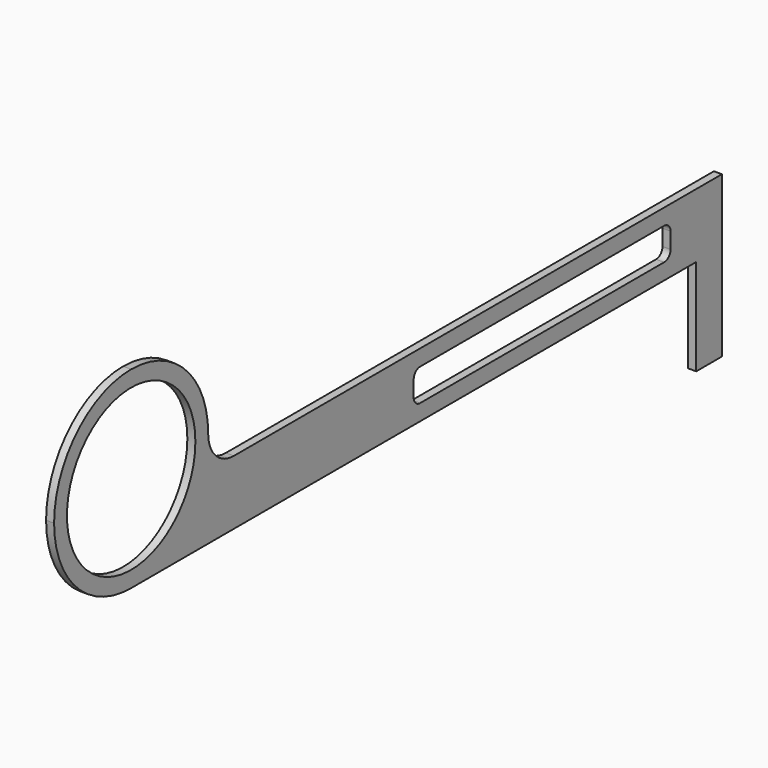
from build123d import *

# Parameters (mm, degrees)
F1_DEPTH = 1.5875
F2_R     = 19.04999
F3_R     = 6.35
F4_R     = 15.875
F5_DEPTH = 25.4
F6_W     = 63.5
F6_H     = 6.35
F7_DEPTH = 25.4
F8_R     = 1.5875


# Not quite as in the source:
# - a fillet or chamfer is up to 0.001 mm smaller than in the source, because OpenCascade refuses the exact size


with BuildPart() as f1:
    # F0 (on Right) → F1 (new body)
    with BuildSketch(Plane.YZ):
        Polygon((-63.1363113923, 43.5325428513), (-101.2363113923, 43.5325428513), (-101.2363113923, 5.4325428513), (57.5136886077, 5.4325428513), (57.5136886077, -13.6174602094), (63.8636886077, -13.6174602094), (63.8636886077, 18.1325428513), (-63.1363113923, 18.1325428513), align=None)
    extrude(amount=F1_DEPTH)

    # F2 (radius 19.05 in the source; OpenCascade refuses exactly that, so slightly less here)
    f2_edges = [f1.edges().sort_by_distance(p)[0] for p in [
        (0.79375, -63.136311, 43.532543),
        (0.79375, -101.236311, 43.532543),
        (0.79375, -101.236311, 5.432543),
    ]]
    fillet(f2_edges, radius=F2_R)

    # F3
    f3_edges = [f1.edges().sort_by_distance(p)[0] for p in [
        (0.79375, -63.136311, 18.132543),
    ]]
    fillet(f3_edges, radius=F3_R)

    # F4 (on face) → F5 (cut)
    with BuildSketch(Plane.YZ.offset(1.5875)):
        with Locations((-82.1863113923, 24.4825428513)):
            Circle(F4_R)
    extrude(amount=-F5_DEPTH, mode=Mode.SUBTRACT)

    # F6 (on face) → F7 (cut)
    with BuildSketch(Plane.YZ.offset(1.5875)):
        with Locations((19.4136886077, 11.7825428513)):
            Rectangle(F6_W, F6_H)
    extrude(amount=-F7_DEPTH, mode=Mode.SUBTRACT)

    # F8
    f8_edges = [f1.edges().sort_by_distance(p)[0] for p in [
        (0.79375, -12.336311, 14.957543),
        (0.79375, -12.336311, 8.607543),
        (0.79375, 51.163689, 8.607543),
        (0.79375, 51.163689, 14.957543),
    ]]
    fillet(f8_edges, radius=F8_R)


solid = f1.part
